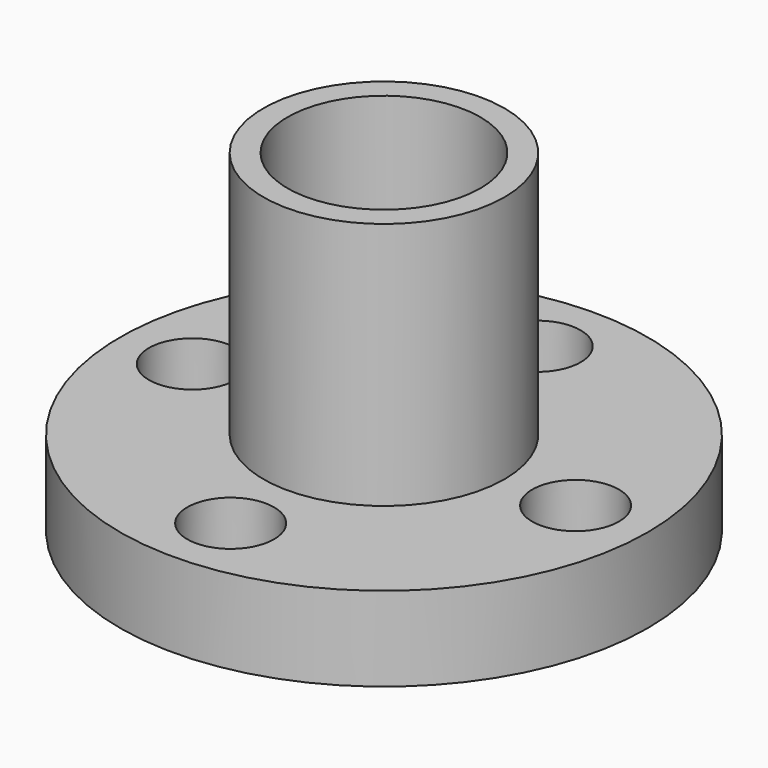
from build123d import *

# Parameters (mm, degrees)
F0_R     = 10.95
F0_R_2   = 1.8
F0_R_3   = 5
F1_DEPTH = 3.5
F0_R_4   = 4
F2_DEPTH = 13.8
F3_DEPTH = 1.5


with BuildPart() as f1:
    # F0 (on Top) → F1 (new body)
    with BuildSketch(Plane.XY):
        Circle(F0_R)
        with Locations((0, -7.95)):
            Circle(F0_R_2, mode=Mode.SUBTRACT)
        with Locations((-7.95, 0)):
            Circle(F0_R_2, mode=Mode.SUBTRACT)
        Circle(F0_R_3, mode=Mode.SUBTRACT)
        with Locations((7.95, 0)):
            Circle(F0_R_2, mode=Mode.SUBTRACT)
        with Locations((0, 7.95)):
            Circle(F0_R_2, mode=Mode.SUBTRACT)
    extrude(amount=F1_DEPTH)


with BuildPart() as f2:
    # F0 (on Top) → F2 (new body)
    with BuildSketch(Plane.XY):
        Circle(F0_R_3)
        Circle(F0_R_4, mode=Mode.SUBTRACT)
    extrude(amount=F2_DEPTH)

    # F0 (on Top) → F3 (join)
    with BuildSketch(Plane.XY):
        Circle(F0_R_3)
        Circle(F0_R_4, mode=Mode.SUBTRACT)
    extrude(amount=-F3_DEPTH)


solid = Compound([f1.part, f2.part])
